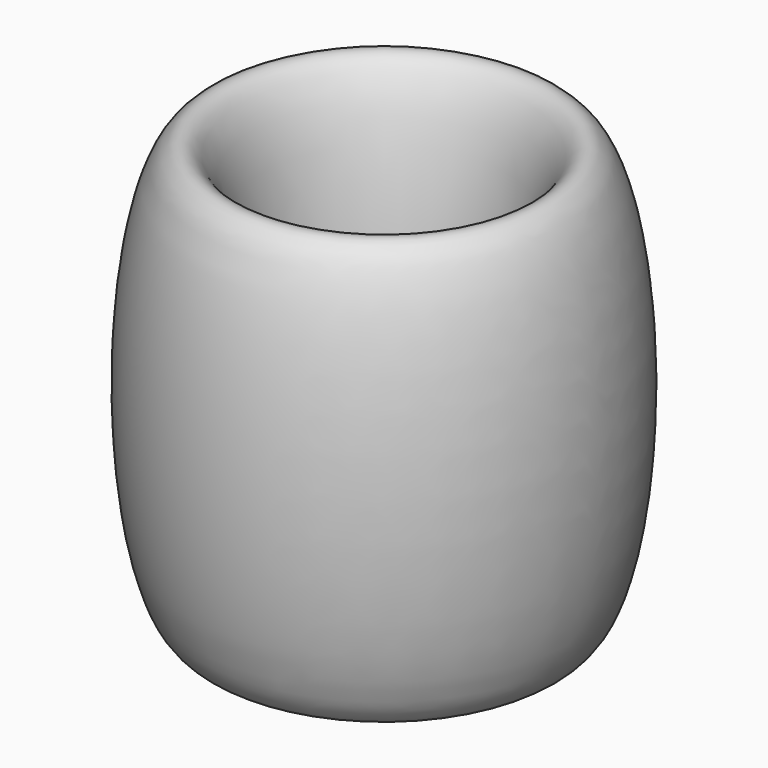
from build123d import *


# Not quite as in the source:
# - a feature names something its author has since deleted; it is built from what else it names


with BuildPart() as f1:
    # F0 (on Front) → F1 (revolve)
    with BuildSketch(Plane.XZ):
        with BuildLine():
            Line((0, 0), (37.5, 0))
            add(Edge.make_bspline(
                [(37.5, 0), (55.0791791491, 0), (49.3069174139, 66.4178932538), (43.5346556788, 132.8357865075), (29.7462116097, 89.2181112443), (15.9577675406, 45.6004359812), (30.7851173902, 7.8269561853)],
                knots=[3.1415926536, 3.1415926536, 3.1415926536, 5.0469534984, 5.0469534984, 6.9523143433, 6.9523143433, 8.8576751881, 8.8576751881, 8.8576751881], degree=2, weights=[1, 0.5795007053, 1, 0.5795007053, 1, 0.5795007053, 1]))
            ThreePointArc((30.7851173902, 7.8269561853), (30.2621170267, 3.1835111332), (26.13084719, 1))
            Line((26.13084719, 1), (0, 1))
            Line((0, 1), (0, 0))
        make_face()
    revolve(axis=Axis((0, 0, 50), (0, 0, 1)))


solid = f1.part
